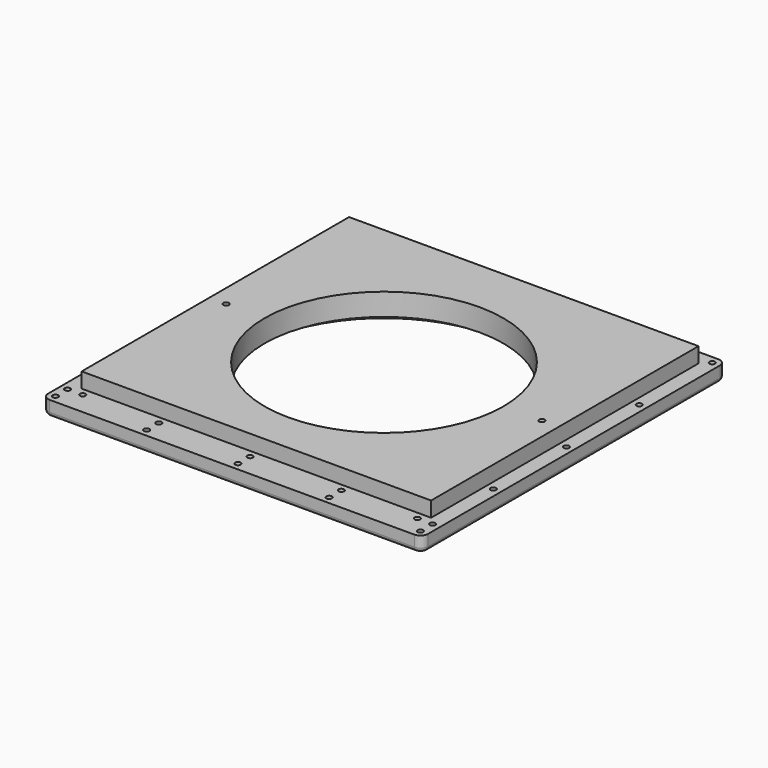
from build123d import *
from build123d import SkipClean  # not in build123d's __all__

# Parameters (mm, degrees)
F0_W           = 450
F0_H           = 18
F1_DEPTH       = 450
F3_D           = 283
F3_DEPTH       = 36
F3_CBORE_D     = 315
F3_CBORE_DEPTH = 9.7
F3_TIP         = 85.0217775924
F4_R           = 9
F5_R           = 5
F7_D           = 6.6
F7_DEPTH       = 6
F7_TIP         = 1.9828400428
F8_ANGLE       = 180
F9_W           = 414
F9_H           = 396
F9_R           = 141.5
F10_DEPTH      = 18
F13_D          = 13.2
F13_DEPTH      = 25
F13_TIP        = 3.9656800856
F14_D          = 6.6
F14_DEPTH      = 6
F14_TIP        = 1.9828400428


# Not quite as in the source:
# - after a boolean that leaves OpenCascade's solid faulty, fix() repairs it


with BuildPart() as f1:
    # F0 (on Front) → F1 (new body)
    with BuildSketch(Plane.XZ):
        with Locations((-0.2429935762, -1.4711191316)):
            Rectangle(F0_W, F0_H)
    extrude(amount=F1_DEPTH)

    # F3
    with Locations(Plane.XY.offset(7.5288808684)):
        with Locations((-0.2429935762, -225)):
            CounterBoreHole(F3_D / 2, F3_CBORE_D / 2, F3_CBORE_DEPTH, depth=F3_DEPTH)
            with Locations((0, 0, -(F3_DEPTH + F3_TIP / 2))):  # 118° drill point
                Cone(0, F3_D / 2, F3_TIP, mode=Mode.SUBTRACT)

    # F4
    f4_edges = [f1.edges().sort_by_distance(p)[0] for p in [
        (-225.242994, -450, -1.471119),
        (-225.242994, 0, -1.471119),
        (224.757006, 0, -1.471119),
        (224.757006, -450, -1.471119),
    ]]
    fillet(f4_edges, radius=F4_R)

    # F5
    f5_edges = [f1.edges().sort_by_distance(p)[0] for p in [
        (-0.242994, 0, 7.528881),
        (224.757006, -225, 7.528881),
        (-0.242994, -450, 7.528881),
        (-225.242994, -225, 7.528881),
    ]]
    fillet(f5_edges, radius=F5_R)

    # F7
    with Locations(Plane(origin=(0, 0, -10.4711191316), x_dir=(1, 0, 0), z_dir=(0, 0, -1))):
        with Locations((-216.2429935762, 441), (-108.1214967881, 441), (0, 441), (108.1214967881, 441), (216.2429935762, 441), (108.1214967881, 423), (0, 423), (-108.1214967881, 423), (-198.2429935762, 423), (198.2429935762, 423), (216.2429935762, 333), (216.2429935762, 225), (216.2429935762, 117), (216.2429935762, 9), (108.1214967881, 9), (0, 9), (-108.1214967881, 9), (-216.2429935762, 9), (-216.2429935762, 117), (-216.2429935762, 225), (-216.2429935762, 333), (-216.2429935762, 423), (216.2429935762, 423)):
            Hole(F7_D / 2, depth=F7_DEPTH)
            with Locations((0, 0, -(F7_DEPTH + F7_TIP / 2))):  # 118° drill point
                Cone(0, F7_D / 2, F7_TIP, mode=Mode.SUBTRACT)


with BuildPart() as f1_1:
    # F8: moved
    add(f1.part.rotate(Axis((224.7570064238, -225, -10.4711191316), (0, 1, 0)), F8_ANGLE), clean=False)

    # F9 (on face) → F10 (join)
    with BuildSketch(Plane.XY.offset(-10.4711191316)):
        with Locations((449.7570064238, -216)):
            Rectangle(F9_W, F9_H)
        with Locations((449.7570064238, -225)):
            Circle(F9_R, mode=Mode.SUBTRACT)
    with SkipClean():  # cleaning this boolean's faces spoils the solid; the shape is the same uncleaned
        extrude(amount=F10_DEPTH)

    # F13
    with Locations(Plane(origin=(0, 0, -28.4711191316), x_dir=(1, 0, 0), z_dir=(0, 0, -1))):
        with Locations((628.2570064238, 46.5), (271.2570064238, 46.5), (271.2570064238, 403.5), (628.2570064238, 403.5)):
            Hole(F13_D / 2, depth=F13_DEPTH)
            with Locations((0, 0, -(F13_DEPTH + F13_TIP / 2))):  # 118° drill point
                Cone(0, F13_D / 2, F13_TIP, mode=Mode.SUBTRACT)

    add(f1_1.part.fix(), mode=Mode.REPLACE)

    # F14
    with Locations(Plane.XY.offset(7.5288808684)):
        with Locations((262.7570064238, -225), (636.7570064238, -225)):
            Hole(F14_D / 2, depth=F14_DEPTH)
            with Locations((0, 0, -(F14_DEPTH + F14_TIP / 2))):  # 118° drill point
                Cone(0, F14_D / 2, F14_TIP, mode=Mode.SUBTRACT)


solid = f1_1.part
